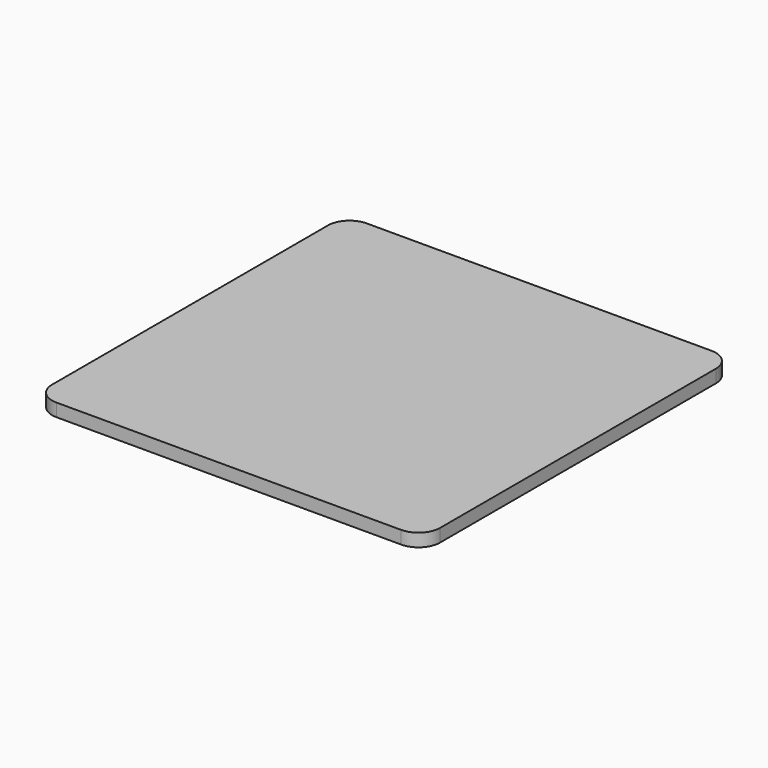
from build123d import *

# Parameters (mm, degrees)
F0_W     = 90
F0_H     = 90
F1_DEPTH = 3
F2_R     = 5


# Not quite as in the source:
# - a feature of the source that left no trace in its solid (it failed there, or was rolled back) is left out


with BuildPart() as f1:
    # F0 (on Top) → F1 (new body)
    with BuildSketch(Plane.XY):
        with Locations((-0.9914580733, 2.9022350864)):
            Rectangle(F0_W, F0_H)
    extrude(amount=-F1_DEPTH)

    # F2
    f2_edges = [f1.edges().sort_by_distance(p)[0] for p in [
        (-45.991458, 47.902235, -1.5),
        (44.008542, 47.902235, -1.5),
        (-45.991458, -42.097765, -1.5),
        (44.008542, -42.097765, -1.5),
    ]]
    fillet(f2_edges, radius=F2_R)


solid = f1.part
